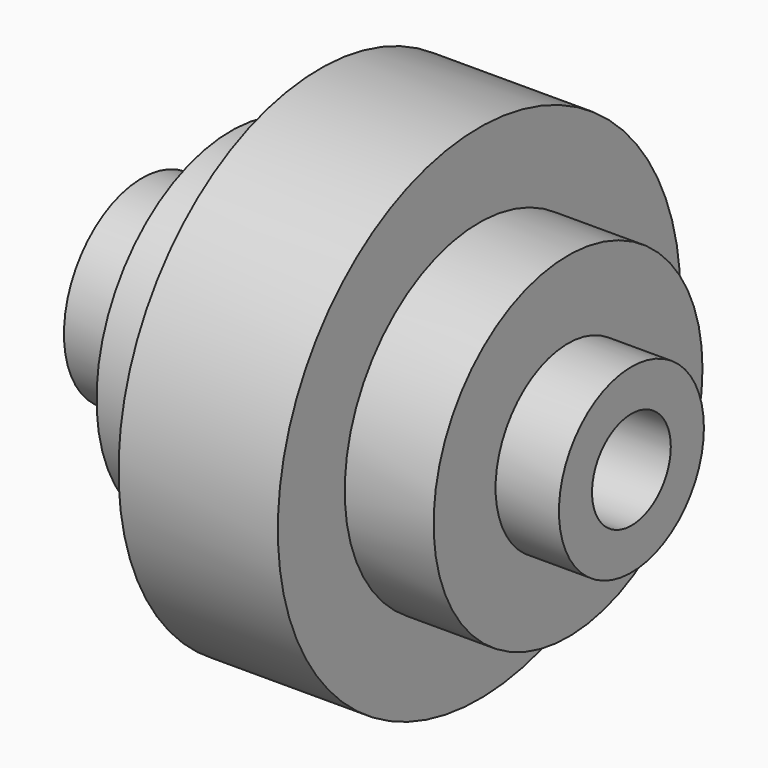
from build123d import *


# Not quite as in the source:
# - the program builds the solid bodies; features that only make, move or delete a surface that nothing else refers to are left out


with BuildPart() as f5:
    # F4 (on Top) → F5 (revolve)
    with BuildSketch(Plane.XY):
        Polygon((-153.7197083235, 10.5134751648), (-49.2208898067, 10.5134751648), (-49.2208898067, 19.3470064551), (-62.753111124, 19.3470064551), (-62.753111124, 35.886388272), (-81.735804677, 35.886388272), (-81.735804677, 53.7413991988), (-115.7543063164, 53.7413991988), (-115.7543063164, 35.886388272), (-134.7369998693, 35.886388272), (-134.7369998693, 20.8505876362), (-153.7197083235, 20.8505876362), align=None)
    revolve(axis=Axis((-106.8370621651, 0, 0), (-1, 0, 0)))


solid = f5.part
